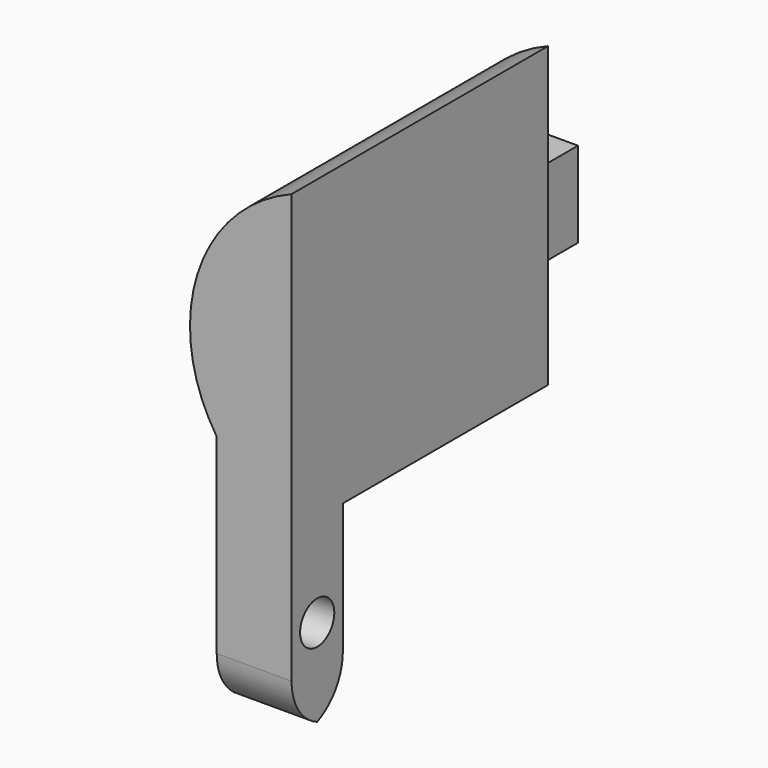
from build123d import *

# Parameters (mm, degrees)
F1_DEPTH    = 19.05
F3_DEPTH    = 2.54
F5_DEPTH    = 4.445
F6_R        = 1.27
F7_DEPTH    = 25.4
F8_T1_DEPTH = 20.32


# Not quite as in the source:
# - a fillet or chamfer that OpenCascade refuses, or shapes differently, is made with other operations: its cross-section is extruded or revolved along the edge and cut away or added


with BuildPart() as f1:
    # F0 (on Front) → F1 (new body)
    with BuildSketch(Plane.XZ):
        with BuildLine():
            Line((-3.4925, 0), (-3.4925, 8.861606443))
            ThreePointArc((-3.4925, 8.861606443), (-9.525, 0), (-3.4925, -8.861606443))
            Line((-3.4925, -8.861606443), (-3.4925, 0))
        make_face()
    extrude(amount=F1_DEPTH)

    # F2 (on face) → F3 (join)
    with BuildSketch(Plane(origin=(0, 0, 0), x_dir=(-1, 0, 0), z_dir=(0, 1, 0))):
        Polygon((3.7465, 2.54), (3.7465, 0), (3.7465, -2.54), (8.8265, -2.54), (8.8265, 2.54), align=None)
    extrude(amount=F3_DEPTH)

    # F4 (on face) → F5 (join)
    with BuildSketch(Plane.YZ.offset(-3.4925)):
        Polygon((-19.05, -2.0384269301), (-19.05, -8.861606443), (-19.05, -19.779715687), (-15.24, -19.779715687), (-15.24, -8.861606443), (-15.24, -2.0384269301), align=None)
    extrude(amount=-F5_DEPTH)

    # F6 (on face) → F7 (cut)
    with BuildSketch(Plane.YZ.offset(-3.4925)):
        with Locations((-17.145, -14.320661065)):
            Circle(F6_R)
    extrude(amount=-F7_DEPTH, mode=Mode.SUBTRACT)

    # F8: fillet of radius 3.175 on 2 edges, made by hand

    # F8_s2 → F8_t1 (cut)
    with BuildSketch(Plane.YZ.offset(-15.875)):
        with BuildLine():
            ThreePointArc((-15.24, -16.604715687), (-16.1699359697, -18.8497797173), (-18.415, -19.779715687))
            Line((-18.415, -19.779715687), (-15.24, -19.779715687))
            Line((-15.24, -19.779715687), (-15.24, -16.604715687))
        make_face()
        with BuildLine():
            ThreePointArc((-19.05, -16.604715687), (-18.1200640303, -18.8497797173), (-15.875, -19.779715687))
            Line((-15.875, -19.779715687), (-19.05, -19.779715687))
            Line((-19.05, -19.779715687), (-19.05, -16.604715687))
        make_face()
    extrude(amount=F8_T1_DEPTH, mode=Mode.SUBTRACT)


solid = f1.part
